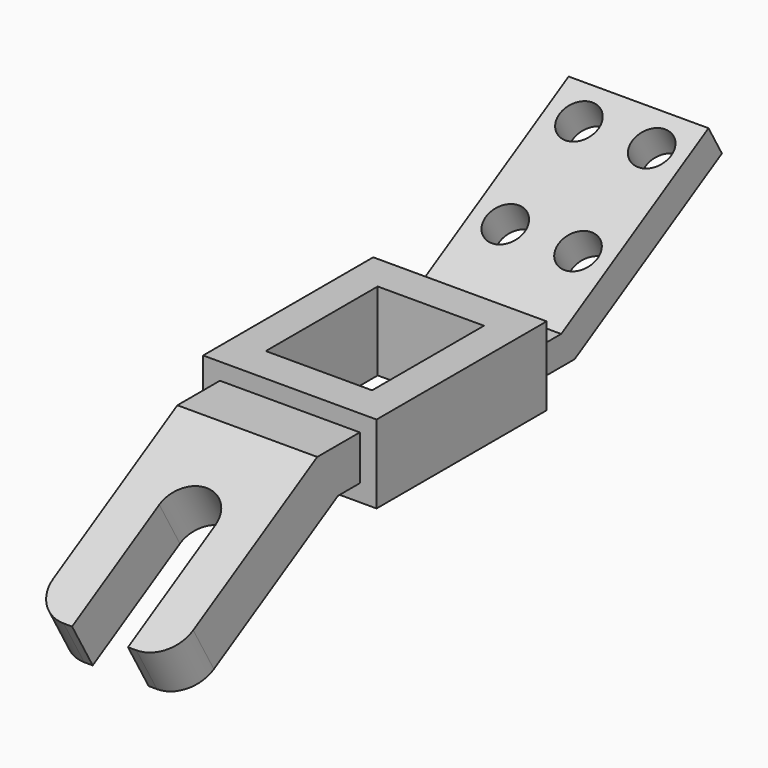
from build123d import *

# Parameters (mm, degrees)
F1_DEPTH = 31
F2_DEPTH = 25
F4_DEPTH = 137.1753371482
F5_R     = 12
F6_R     = 7
F7_DEPTH = 77.8189306876
F8_W     = 38
F8_H     = 50
F9_DEPTH = 60.001


# Not quite as in the source:
# - a feature of the source that left no trace in its solid (it failed there, or was rolled back) is left out


with BuildPart() as f1:
    # F0 (on Right) → F1 (new body, symmetric)
    with BuildSketch(Plane.YZ):
        Polygon((38, 2.3923048454), (38, 14), (-38, 14), (-38, 8), (-38, -8), (-38, -14), (38, -14), (38, -8), align=None)
    extrude(amount=F1_DEPTH, both=True)

    # F0 (on Right) → F2 (join, symmetric)
    with BuildSketch(Plane.YZ):
        Polygon((-38, -8), (-38, 8), (-57, 8), (-122.8179306876, -30), (-113.5803263806, -46), (-47.762395693, -8), align=None)
        Polygon((52, 2.3923048454), (38, 2.3923048454), (38, -8), (58, -8), (123.8179306876, 30), (117.8179306876, 40.3923048454), align=None)
    extrude(amount=F2_DEPTH, both=True)

    # F3 (on face) → F4 (cut, through all)
    with BuildSketch(Plane(origin=(0, -17.7141016151, 30.6817240079), x_dir=(1, 0, 0), z_dir=(0, -0.5, 0.8660254038))):
        with BuildLine():
            Line((10, -121.3634480157), (10, -76.3634480157))
            ThreePointArc((10, -76.3634480157), (0, -86.3634480157), (-10, -76.3634480157))
            Line((-10, -76.3634480157), (-10, -121.3634480157))
            Line((-10, -121.3634480157), (10, -121.3634480157))
        make_face()
        with BuildLine():
            ThreePointArc((-10, -76.3634480157), (0, -86.3634480157), (10, -76.3634480157))
            ThreePointArc((10, -76.3634480157), (0, -66.3634480157), (-10, -76.3634480157))
        make_face()
    extrude(amount=-F4_DEPTH, mode=Mode.SUBTRACT)

    # F5
    f5_edges = [f1.edges().sort_by_distance(p)[0] for p in [
        (25, -118.199129, -38),
        (-25, -118.199129, -38),
    ]]
    fillet(f5_edges, radius=F5_R)

    # F6 (on face) → F7 (cut, through all)
    with BuildSketch(Plane(origin=(0, 11.9641016151, -20.7224318643), x_dir=(1, 0, 0), z_dir=(0, -0.5, 0.8660254038))):
        with Locations((-13, 110.2294734195)):
            Circle(F6_R)
        with Locations((13, 110.2294734195)):
            Circle(F6_R)
        with Locations((13, 72.2294734195)):
            Circle(F6_R)
        with Locations((-13, 72.2294734195)):
            Circle(F6_R)
    extrude(amount=-F7_DEPTH, mode=Mode.SUBTRACT)

    # F8 (on face) → F9 (cut, through all)
    with BuildSketch(Plane.XY.offset(14)):
        Rectangle(F8_W, F8_H)
    extrude(amount=-F9_DEPTH, mode=Mode.SUBTRACT)


solid = f1.part
